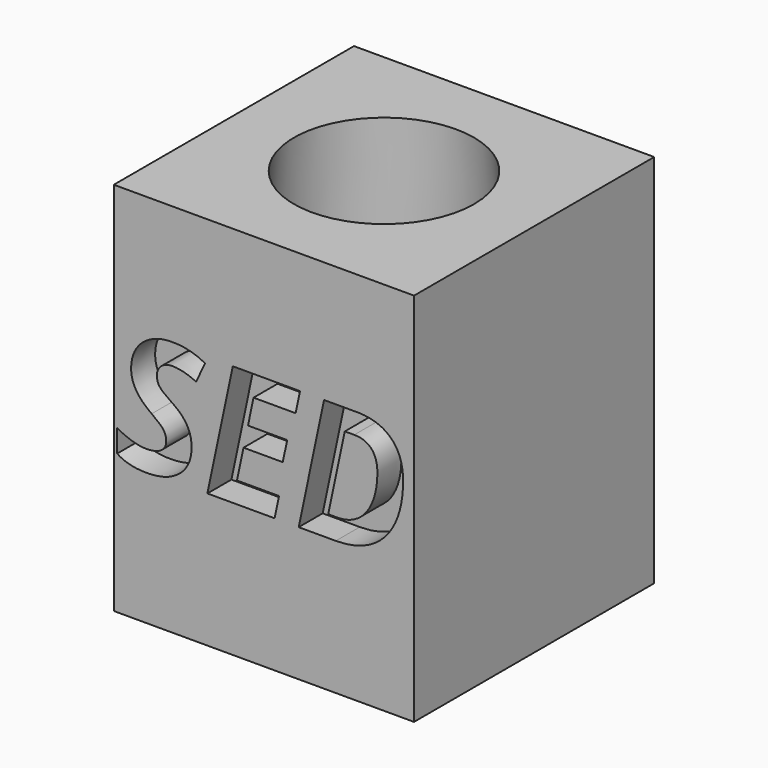
from build123d import *

# Parameters (mm, degrees)
F0_W         = 25.4
F0_H         = 25.4
F1_DEPTH     = 31.75
F2_R         = 7.62
F3_DEPTH     = 31.75
F3_TAPER     = -3
F4_TEXT_SIZE = 14.2484003857
F5_DEPTH     = 2.54


# Not quite as in the source:
# - Text() gives the source's letters only with a copy of the font that has no kerning and outlines rounded to 1/6400 em; it was checked with that copy


with BuildPart() as f1:
    # F0 (on Top) → F1 (new body)
    with BuildSketch(Plane.XY):
        with Locations((12.7, 12.7)):
            Rectangle(F0_W, F0_H)
    extrude(amount=F1_DEPTH)

    # F2 (on face) → F3 (cut)
    with BuildSketch(Plane.XY.offset(31.75)):
        with Locations((12.7, 12.7)):
            Circle(F2_R)
    extrude(amount=-F3_DEPTH, taper=F3_TAPER, mode=Mode.SUBTRACT)

    # F4 (on face) → F5 (cut)
    with BuildSketch(Plane.XZ):
        with Locations((0, 11.3311517223)):
            Text('SED', F4_TEXT_SIZE, font='Open Sans', font_style=FontStyle.BOLDITALIC, text_align=(TextAlign.LEFT, TextAlign.BOTTOM))
    extrude(amount=-F5_DEPTH, mode=Mode.SUBTRACT)


solid = f1.part
